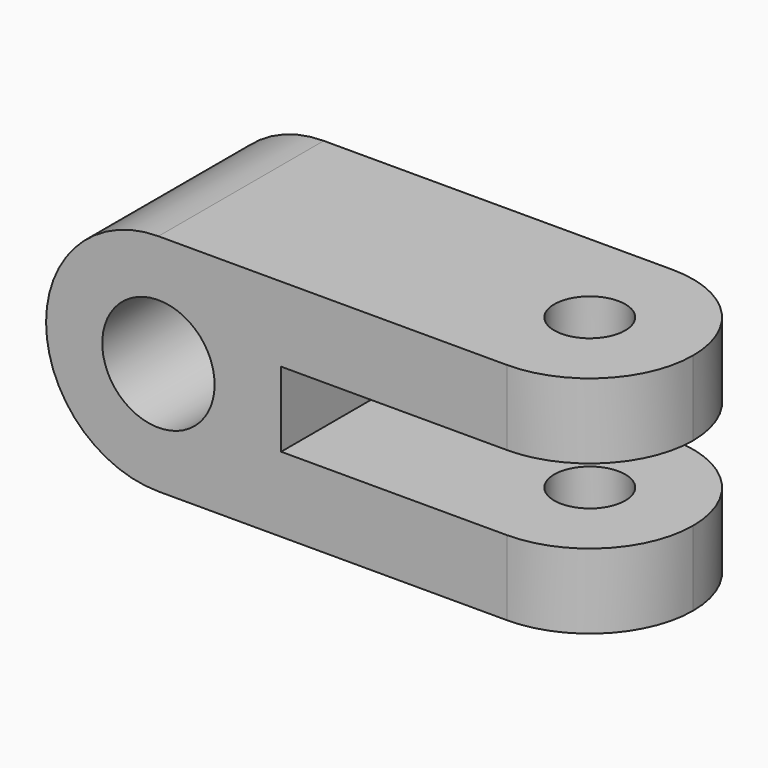
from build123d import *

# Parameters (mm, degrees)
F0_R     = 6.985
F2_DEPTH = 44.196
F1_R     = 11.049
F3_DEPTH = 40.641
F4_R     = 22.098
F5_R     = 22.09799
F1_W     = 64.77
F1_H     = 14.732
F6_DEPTH = 40.641


# Not quite as in the source:
# - a fillet or chamfer is up to 0.001 mm smaller than in the source, because OpenCascade refuses the exact size


with BuildPart() as f2:
    # F0 (on Top) → F2 (new body)
    with BuildSketch(Plane.XY):
        with BuildLine():
            Line((0, 40.64), (0, 0))
            Line((0, 0), (90.678, 0))
            ThreePointArc((90.678, 0), (70.358, 20.32), (90.678, 40.64))
            Line((90.678, 40.64), (0, 40.64))
        make_face()
        with BuildLine():
            ThreePointArc((90.678, 40.64), (70.358, 20.32), (90.678, 0))
            ThreePointArc((90.678, 0), (105.0464097937, 5.9515902063), (110.998, 20.32))
            ThreePointArc((110.998, 20.32), (105.0464097937, 34.6884097937), (90.678, 40.64))
        make_face()
        with Locations((90.678, 20.32)):
            Circle(F0_R, mode=Mode.SUBTRACT)
    extrude(amount=F2_DEPTH)

    # F1 (on Front) → F3 (cut, through all)
    with BuildSketch(Plane.XZ):
        with Locations((22.098, 22.098)):
            Circle(F1_R)
    extrude(amount=-F3_DEPTH, mode=Mode.SUBTRACT)

    # F4
    f4_edges = [f2.edges().sort_by_distance(p)[0] for p in [
        (0, 20.32, 44.196),
    ]]
    fillet(f4_edges, radius=F4_R)

    # F5 (radius 22.098 in the source; OpenCascade refuses exactly that, so slightly less here)
    f5_edges = [f2.edges().sort_by_distance(p)[0] for p in [
        (0, 20.32, 0),
    ]]
    fillet(f5_edges, radius=F5_R)

    # F1 (on Front) → F6 (cut, through all)
    with BuildSketch(Plane.XZ):
        with Locations((78.613, 22.098)):
            Rectangle(F1_W, F1_H)
    extrude(amount=-F6_DEPTH, mode=Mode.SUBTRACT)


solid = f2.part
